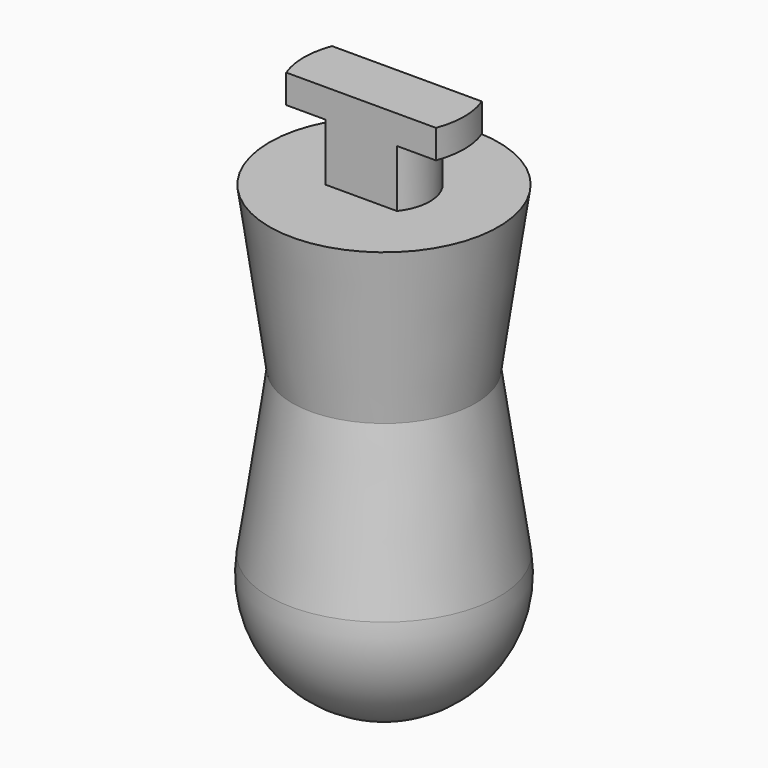
from build123d import *

# Parameters (mm, degrees)
F3_DEPTH = 9.525


with BuildPart() as f1:
    # F0 (on Front) → F1 (revolve)
    with BuildSketch(Plane.XZ):
        Polygon((0, -18.0305813839), (0, 0), (-5.08, 0), (-12.7, 0), (-10.16, -18.0305813839), align=None)
        Polygon((-5.08, 0), (0, 0), (0, 9.525), (-8.89, 9.525), (-8.89, 6.35), (-5.08, 6.35), align=None)
        Polygon((0, -36.0611627679), (0, -18.0305813839), (-10.16, -18.0305813839), (-12.7635, -36.0611627679), align=None)
        with BuildLine():
            Line((0, -50.8), (0, -36.0611627679))
            Line((0, -36.0611627679), (-12.7635, -36.0611627679))
            ThreePointArc((-12.7635, -36.0611627679), (-9.7485929139, -46.3461912692), (0, -50.8))
        make_face()
    revolve(axis=Axis((0, 0, -25.4), (0, 0, -1)))

    # F2 (on face) → F3 (cut, through all)
    with BuildSketch(Plane.XY.offset(9.525)):
        with BuildLine():
            ThreePointArc((8.3037024874, 3.175), (0, 8.89), (-8.3037024874, 3.175))
            Line((-8.3037024874, 3.175), (8.3037024874, 3.175))
        make_face()
        with BuildLine():
            Line((8.3037024874, -3.175), (-8.3037024874, -3.175))
            ThreePointArc((-8.3037024874, -3.175), (0, -8.89), (8.3037024874, -3.175))
        make_face()
        with BuildLine():
            ThreePointArc((10.9695693512, 3.175), (0, 11.4198107144), (-10.9695693512, 3.175))
            Line((-10.9695693512, 3.175), (-8.3037024874, 3.175))
            ThreePointArc((-8.3037024874, 3.175), (0, 8.89), (8.3037024874, 3.175))
            Line((8.3037024874, 3.175), (10.9695693512, 3.175))
        make_face()
        with BuildLine():
            Line((-8.3037024874, -3.175), (-10.9695693512, -3.175))
            ThreePointArc((-10.9695693512, -3.175), (0, -11.4198107144), (10.9695693512, -3.175))
            Line((10.9695693512, -3.175), (8.3037024874, -3.175))
            ThreePointArc((8.3037024874, -3.175), (0, -8.89), (-8.3037024874, -3.175))
        make_face()
        with BuildLine():
            Line((-8.3037024874, 3.175), (-10.9695693512, 3.175))
            ThreePointArc((-10.9695693512, 3.175), (-11.4198107144, 0), (-10.9695693512, -3.175))
            Line((-10.9695693512, -3.175), (-8.3037024874, -3.175))
            ThreePointArc((-8.3037024874, -3.175), (-8.89, 0), (-8.3037024874, 3.175))
        make_face()
        with BuildLine():
            ThreePointArc((11.4198107144, 0), (11.3066901072, 1.6033825405), (10.9695693512, 3.175))
            Line((10.9695693512, 3.175), (8.3037024874, 3.175))
            ThreePointArc((8.3037024874, 3.175), (8.7421969525, 1.6143396307), (8.89, 0))
            ThreePointArc((8.89, 0), (8.7421969525, -1.6143396307), (8.3037024874, -3.175))
            Line((8.3037024874, -3.175), (10.9695693512, -3.175))
            ThreePointArc((10.9695693512, -3.175), (11.3066901072, -1.6033825405), (11.4198107144, 0))
        make_face()
    extrude(amount=-F3_DEPTH, mode=Mode.SUBTRACT)


solid = f1.part
